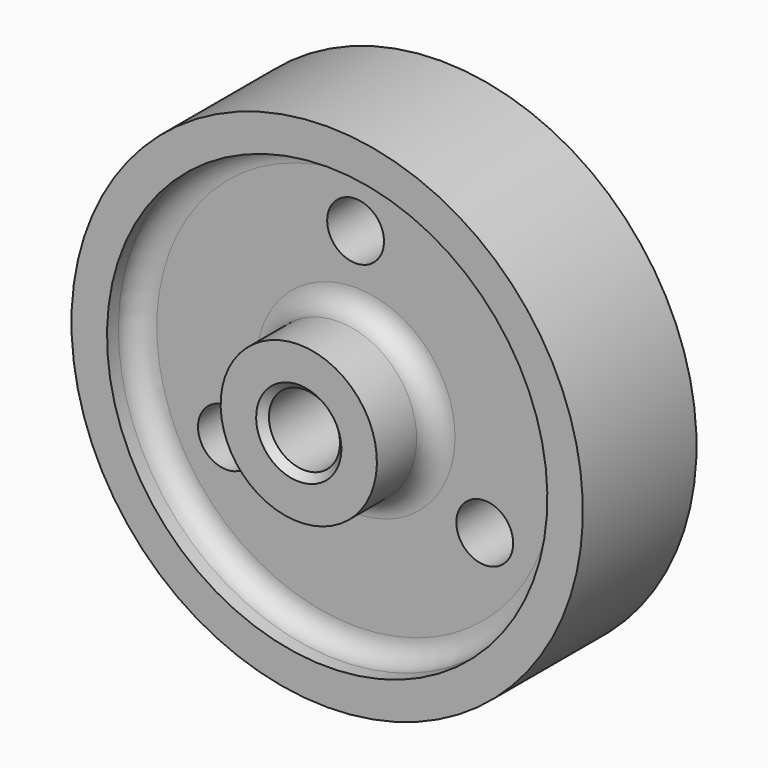
from build123d import *

# Parameters (mm, degrees)
F2_SIZE         = 1
F3_R            = 4
F4_DEPTH        = 15
F4_COPIES_COUNT = 3
F6_D            = 4
F6_DEPTH        = 12
F6_TIP          = 1.2017212381


# Not quite as in the source:
# - a pattern or mirror of a feature is missing from the dataset's text; its kind, count and spacing are read off the source's solid


with BuildPart() as f1:
    # F0 (on Right) → F1 (revolve)
    with BuildSketch(Plane.YZ):
        with BuildLine():
            Line((0, 11), (0, 5))
            Line((0, 5), (25, 5))
            Line((25, 5), (25, 36))
            Line((25, 36), (5, 36))
            Line((5, 36), (5, 31))
            Line((5, 31), (7, 31))
            ThreePointArc((7, 31), (9.1213203436, 30.1213203436), (10, 28))
            Line((10, 28), (10, 14))
            ThreePointArc((10, 14), (9.1213203436, 11.8786796564), (7, 11))
            Line((7, 11), (0, 11))
        make_face()
    revolve(axis=Axis((0, 9.0291841974, 0), (0, 1, 0)))

    # F2
    f2_edges = [f1.edges().sort_by_distance(p)[0] for p in [
        (0, 0, -5),
    ]]
    chamfer(f2_edges, length=F2_SIZE)

    # F3 (on face) → F4 (cut, through all)
    with BuildSketch(Plane(origin=(0, 25, 0), x_dir=(-1, 0, 0), z_dir=(0, 1, 0))):
        with Locations((0, 21)):
            Circle(F3_R)
    f4 = extrude(amount=-F4_DEPTH, mode=Mode.SUBTRACT)

    # F4_copies: F4 ×3 about axis
    f4_copies_axis = Axis((0, 0, 0), (0, 1, 0))
    for i in range(1, F4_COPIES_COUNT):
        add(f4.rotate(f4_copies_axis, i * 360 / F4_COPIES_COUNT), mode=Mode.SUBTRACT)

    # F6
    with Locations(Plane(origin=(0, 25, 0), x_dir=(-1, 0, 0), z_dir=(0, 1, 0))):
        with Locations((0, 5)):
            Hole(F6_D / 2, depth=F6_DEPTH)
            with Locations((0, 0, -(F6_DEPTH + F6_TIP / 2))):  # 118° drill point
                Cone(0, F6_D / 2, F6_TIP, mode=Mode.SUBTRACT)


solid = f1.part
